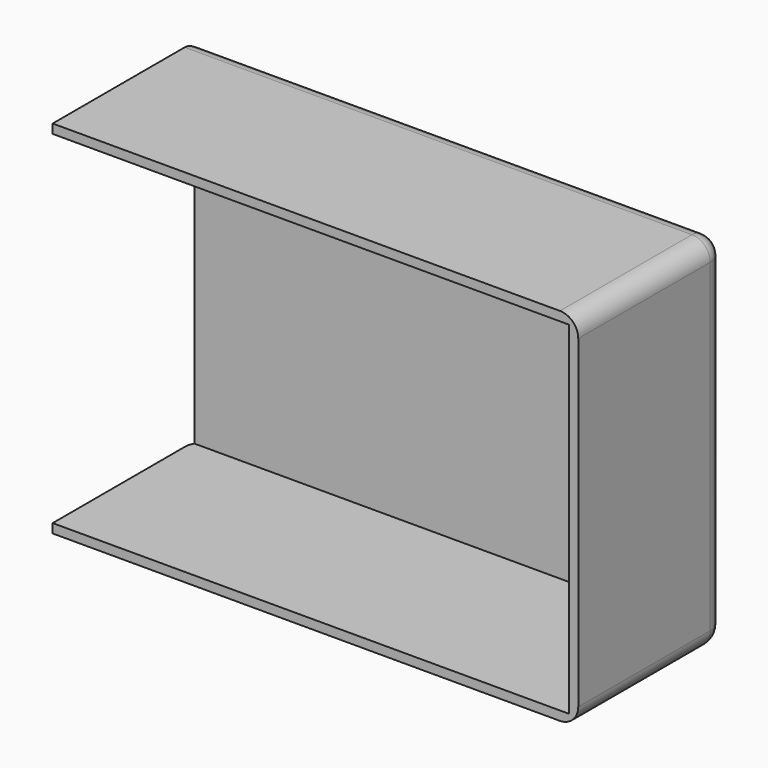
from build123d import *

# Parameters (mm, degrees)
F0_W         = 145.6760466099
F0_H         = 100.0369116664
F0_W_2       = 138.8105116785
F0_H_2       = 92.9268449545
F1_DEPTH     = 25.4
F2_T         = -2.54
F3_T1_DEPTH  = 171.0760466099
F3_T3_DEPTH  = 125.4369116664
F4_DEPTH     = 25.4
F5_T1_DEPTH  = 58.42
F5_S5_W      = 5.08
F5_S5_H      = 5.08
F5_T6_DEPTH  = 5.08
F5_S11_W     = 5.08
F5_S11_H     = 5.08
F5_T12_DEPTH = 5.08


# Not quite as in the source:
# - a fillet or chamfer that OpenCascade refuses, or shapes differently, is made with other operations: its cross-section is extruded or revolved along the edge and cut away or added


with BuildPart() as f1:
    # F0 (on Front) → F1 (new body)
    with BuildSketch(Plane.XZ):
        with Locations((-20.1583206654, 2.9303953052)):
            Rectangle(F0_W, F0_H)
        with Locations((-20.7056272775, 3.0381605029)):
            Rectangle(F0_W_2, F0_H_2, mode=Mode.SUBTRACT)
        with Locations((-20.7056272775, 3.0381605029)):
            Rectangle(F0_W_2, F0_H_2)
    extrude(amount=F1_DEPTH)

    # F2
    f2_openings = [f1.faces().sort_by_distance(p)[0] for p in [
        (-20.158321, -25.4, 2.930395),
        (-92.996344, -12.7, 2.930395),
    ]]
    offset(amount=F2_T, openings=f2_openings)

    # F3: fillet of radius 5.08 on 4 edges, made by hand

    # F3_s2 → F3_t1 (cut)
    with BuildSketch(Plane.YZ.offset(-105.6963439703)):
        with BuildLine():
            ThreePointArc((-5.08, 52.9488511384), (-1.4878975516, 51.4609535868), (0, 47.8688511384))
            Line((0, 47.8688511384), (0, 52.9488511384))
            Line((0, 52.9488511384), (-5.08, 52.9488511384))
        make_face()
        with BuildLine():
            ThreePointArc((-5.08, -47.088060528), (-1.4878975516, -45.6001629765), (0, -42.008060528))
            Line((0, -42.008060528), (0, -47.088060528))
            Line((0, -47.088060528), (-5.08, -47.088060528))
        make_face()
    extrude(amount=F3_T1_DEPTH, mode=Mode.SUBTRACT)

    # F3_s4 → F3_t3 (cut)
    with BuildSketch(Plane.XY.offset(-59.788060528)):
        with BuildLine():
            ThreePointArc((-87.9163439703, 0), (-91.5084464187, -1.4878975516), (-92.9963439703, -5.08))
            Line((-92.9963439703, -5.08), (-92.9963439703, 0))
            Line((-92.9963439703, 0), (-87.9163439703, 0))
        make_face()
        with BuildLine():
            ThreePointArc((52.6797026396, -5.08), (51.191805088, -1.4878975516), (47.5997026396, 0))
            Line((47.5997026396, 0), (52.6797026396, 0))
            Line((52.6797026396, 0), (52.6797026396, -5.08))
        make_face()
    extrude(amount=F3_T3_DEPTH, mode=Mode.SUBTRACT)

    # F4 (add): a face of the model
    f4_faces = [f1.faces().sort_by_distance(p)[0] for p in [
        (-20.1583206654, -25.4, 51.1816812469),
    ]]
    extrude(f4_faces, amount=F4_DEPTH)

    # F5: fillet of radius 5.08 on 2 edges, made by hand

    # F5_s2 → F5_t1 (cut)
    with BuildSketch(Plane.XZ.offset(5.08)):
        with BuildLine():
            ThreePointArc((52.6797026396, 47.8688511384), (51.191805088, 51.4609535868), (47.5997026396, 52.9488511384))
            Line((47.5997026396, 52.9488511384), (52.6797026396, 52.9488511384))
            Line((52.6797026396, 52.9488511384), (52.6797026396, 47.8688511384))
        make_face()
        with BuildLine():
            ThreePointArc((47.5997026396, -47.088060528), (51.191805088, -45.6001629765), (52.6797026396, -42.008060528))
            Line((52.6797026396, -42.008060528), (52.6797026396, -47.088060528))
            Line((52.6797026396, -47.088060528), (47.5997026396, -47.088060528))
        make_face()
    extrude(amount=F5_T1_DEPTH, mode=Mode.SUBTRACT)


with BuildPart() as f5_tool4:
    # F5_s5 → F5_t6 (new body)
    with BuildSketch(Plane.XY.offset(-42.008060528)):
        with Locations((50.1397026396, -2.54)):
            Rectangle(F5_S5_W, F5_S5_H)
    extrude(amount=-F5_T6_DEPTH)

    # F5_s7 → F5_t8 (revolve, cut)
    with BuildSketch(Plane(origin=(47.5997026396, -5.08, -42.008060528), x_dir=(-0.7071067812, -0.7071067812, 0), z_dir=(0.7071067812, -0.7071067812, 0))):
        with BuildLine():
            ThreePointArc((0, -5.08), (5.08, 0), (0, 5.08))
            Line((0, 5.08), (0, -5.08))
        make_face()
    revolve(axis=Axis((47.5997026396, -5.08, -42.008060528), (0, 0, -1)), mode=Mode.SUBTRACT)


with BuildPart() as f1_1:
    add(f1.part)

    # F5_t3: cut F5_tool4
    add(f5_tool4.part, mode=Mode.SUBTRACT)


with BuildPart() as f5_tool10:
    # F5_s11 → F5_t12 (new body)
    with BuildSketch(Plane.YZ.offset(47.5997026396)):
        with Locations((-2.54, 50.4088511384)):
            Rectangle(F5_S11_W, F5_S11_H)
    extrude(amount=F5_T12_DEPTH)

    # F5_s13 → F5_t14 (revolve, cut)
    with BuildSketch(Plane(origin=(47.5997026396, -5.08, 47.8688511384), x_dir=(0, -0.7071067812, -0.7071067812), z_dir=(0, -0.7071067812, 0.7071067812))):
        with BuildLine():
            ThreePointArc((0, -5.08), (5.08, 0), (0, 5.08))
            Line((0, 5.08), (0, -5.08))
        make_face()
    revolve(axis=Axis((47.5997026396, -5.08, 47.8688511384), (1, 0, 0)), mode=Mode.SUBTRACT)


with BuildPart() as f1_2:
    add(f1_1.part)

    # F5_t9: cut F5_tool10
    add(f5_tool10.part, mode=Mode.SUBTRACT)


solid = f1_2.part
